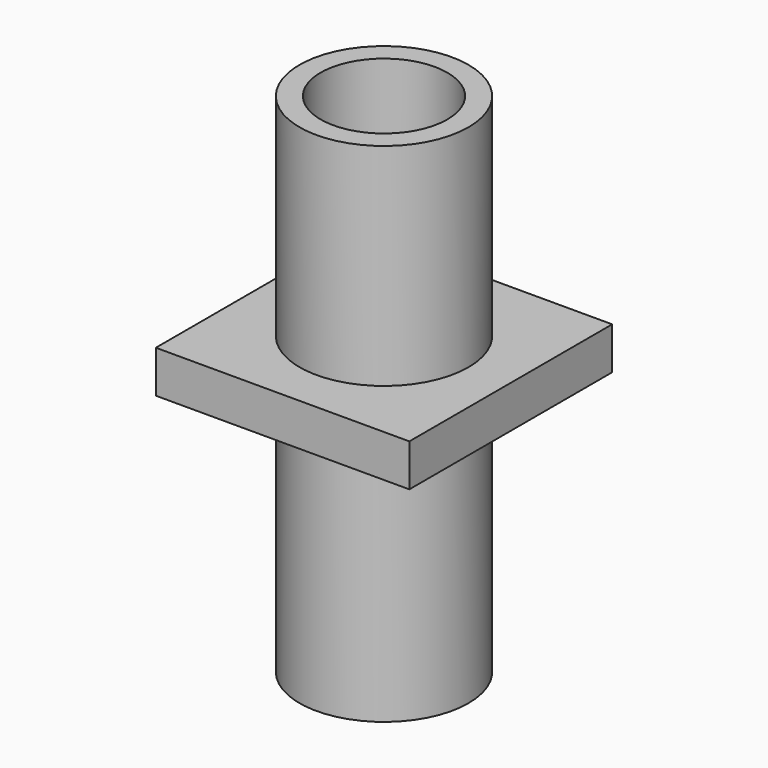
from build123d import *

# Parameters (mm, degrees)
F0_R     = 12.7
F0_R_2   = 9.525
F1_DEPTH = 38.1
F2_W     = 38.1
F2_H     = 38.1
F2_R     = 9.525
F3_DEPTH = 6.35
F4_R     = 12.7
F4_R_2   = 9.525
F5_DEPTH = 38.1


with BuildPart() as f1:
    # F0 (on Top) → F1 (new body)
    with BuildSketch(Plane.XY):
        Circle(F0_R)
        Circle(F0_R_2, mode=Mode.SUBTRACT)
    extrude(amount=F1_DEPTH)

    # F2 (on Top) → F3 (join)
    with BuildSketch(Plane.XY):
        Rectangle(F2_W, F2_H)
        Circle(F2_R, mode=Mode.SUBTRACT)
    extrude(amount=F3_DEPTH)

    # F4 (on face) → F5 (join)
    with BuildSketch(Plane(origin=(0, 0, 0), x_dir=(1, 0, 0), z_dir=(0, 0, -1))):
        Circle(F4_R)
        Circle(F4_R_2, mode=Mode.SUBTRACT)
    extrude(amount=F5_DEPTH)


solid = f1.part
